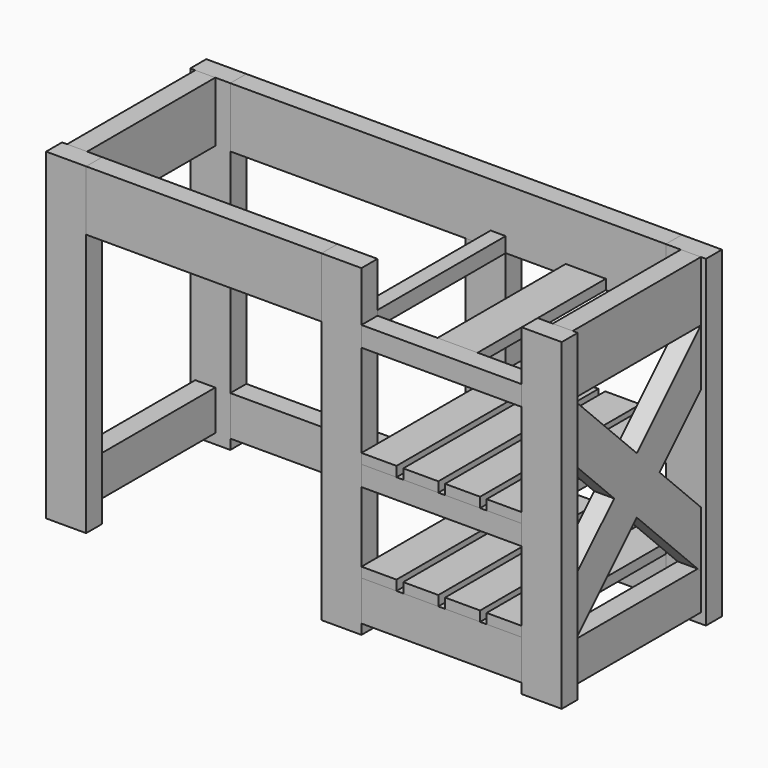
from build123d import *

# Parameters (mm, degrees)
F0_W      = 50.8
F0_H      = 819.15
F1_DEPTH  = 101.6
F2_W      = 50.8
F2_H      = 152.4
F3_DEPTH  = 406.4
F2_H_2    = 101.6
F5_DEPTH  = 50.8
F9_W      = 50.8
F9_H      = 50.8
F10_DEPTH = 406.4
F6_W      = 50.8
F6_H      = 101.6
F12_DEPTH = 1104.9
F11_W     = 50.8
F11_H     = 819.15
F13_DEPTH = 101.6
F11_H_2   = 539.75
F14_W     = 88.9
F14_H     = 25.4
F15_DEPTH = 508
F16_DEPTH = 406.4
F17_W     = 50.8
F17_H     = 152.4
F18_DEPTH = 596.9
F19_DEPTH = 1104.9
F20_W     = 101.6
F20_H     = 25.4
F21_DEPTH = 406.4
F20_W_2   = 38.0999999999
F20_H_2   = 38.1
F20_W_3   = 38.1


# Not quite as in the source:
# - a feature names something its author has since deleted; it is built from what else it names


with BuildPart() as f1:
    # F0 (on Right) → F1 (new body)
    with BuildSketch(Plane.YZ):
        with Locations((-228.6, 0)):
            Rectangle(F0_W, F0_H)
    extrude(amount=F1_DEPTH)


with BuildPart() as f1b:
    # F0 (on Right) → F1, piece 2 (new body)
    with BuildSketch(Plane.YZ):
        with Locations((228.6, 0)):
            Rectangle(F0_W, F0_H)
    extrude(amount=F1_DEPTH)


with BuildPart() as f3:
    # F2 (on face) → F3 (new body, through all)
    with BuildSketch(Plane(origin=(0, -203.2, 0), x_dir=(-1, 0, 0), z_dir=(0, 1, 0))):
        with Locations((-63.5, 333.375)):
            Rectangle(F2_W, F2_H)
    extrude(amount=F3_DEPTH)


with BuildPart() as f3b:
    # F2 (on face) → F3, piece 2 (new body, through all)
    with BuildSketch(Plane(origin=(0, -203.2, 0), x_dir=(-1, 0, 0), z_dir=(0, 1, 0))):
        with Locations((-63.5, -333.375)):
            Rectangle(F2_W, F2_H_2)
    extrude(amount=F3_DEPTH)


with BuildPart() as f5:
    # F4 (on face) → F5 (new body)
    with BuildSketch(Plane.YZ.offset(88.9)):
        Polygon((0, 53.975), (-203.2, 257.175), (-203.2, 113.4909020629), (-71.8420489686, -17.8670489685), (0, -89.7090979371), (203.2, -292.9090979371), (203.2, -149.225), (71.8420489685, -17.8670489685), align=None)
        Polygon((203.2, 257.175), (0, 53.975), (71.8420489685, -17.8670489685), (203.2, 113.4909020629), align=None)
        Polygon((0, -89.7090979371), (-71.8420489686, -17.8670489685), (-203.2, -149.225), (-203.2, -292.9090979371), align=None)
    extrude(amount=-F5_DEPTH)


with BuildPart() as f8_1:
    # F8: instance of F1b
    add(f1b.part.mirror(Plane(origin=(-552.45, -228.6, 0), x_dir=(0, 1, 0), z_dir=(-1, 0, 0))))


with BuildPart() as f8_2:
    # F8: instance of F3
    add(f3.part.mirror(Plane(origin=(-552.45, -228.6, 0), x_dir=(0, 1, 0), z_dir=(-1, 0, 0))))


with BuildPart() as f8_3:
    # F8: instance of F1
    add(f1.part.mirror(Plane(origin=(-552.45, -228.6, 0), x_dir=(0, 1, 0), z_dir=(-1, 0, 0))))


with BuildPart() as f8_4:
    # F8: instance of F3b
    add(f3b.part.mirror(Plane(origin=(-552.45, -228.6, 0), x_dir=(0, 1, 0), z_dir=(-1, 0, 0))))


with BuildPart() as f10:
    # F9 (on face) → F10 (new body)
    with BuildSketch(Plane(origin=(0, 0, 0), x_dir=(0, -1, 0), z_dir=(-1, 0, 0))):
        with Locations((228.6, 257.175)):
            Rectangle(F9_W, F9_H)
    extrude(amount=F10_DEPTH)


with BuildPart() as f10b:
    # F9 (on face) → F10, piece 2 (new body)
    with BuildSketch(Plane(origin=(0, 0, 0), x_dir=(0, -1, 0), z_dir=(-1, 0, 0))):
        with Locations((228.6, -53.975)):
            Rectangle(F9_W, F9_H)
    extrude(amount=F10_DEPTH)


with BuildPart() as f10c:
    # F9 (on face) → F10, piece 3 (new body)
    with BuildSketch(Plane(origin=(0, 0, 0), x_dir=(0, -1, 0), z_dir=(-1, 0, 0))):
        with Locations((-228.6, -53.975)):
            Rectangle(F9_W, F9_H)
    extrude(amount=F10_DEPTH)


with BuildPart() as f12:
    # F6 (on face) → F12 (new body, through all)
    with BuildSketch(Plane(origin=(0, 0, 0), x_dir=(0, -1, 0), z_dir=(-1, 0, 0))):
        with Locations((-228.6, -333.375)):
            Rectangle(F6_W, F6_H)
    extrude(amount=F12_DEPTH)


with BuildPart() as f13:
    # F11 (on face) → F13 (new body)
    with BuildSketch(Plane(origin=(-406.4, 0, 0), x_dir=(0, -1, 0), z_dir=(-1, 0, 0))):
        with Locations((228.6, 0)):
            Rectangle(F11_W, F11_H)
    extrude(amount=F13_DEPTH)


with BuildPart() as f13b:
    # F11 (on face) → F13, piece 2 (new body)
    with BuildSketch(Plane(origin=(-406.4, 0, 0), x_dir=(0, -1, 0), z_dir=(-1, 0, 0))):
        with Locations((-228.6, -12.7)):
            Rectangle(F11_W, F11_H_2)
    extrude(amount=F13_DEPTH)


with BuildPart() as f15:
    # F14 (on face) → F15 (new body, through all)
    with BuildSketch(Plane.XZ.offset(254)):
        with Locations((-44.45, -15.875)):
            Rectangle(F14_W, F14_H)
    extrude(amount=-F15_DEPTH)


with BuildPart() as f15b:
    # F14 (on face) → F15, piece 2 (new body, through all)
    with BuildSketch(Plane.XZ.offset(254)):
        with Locations((-361.95, -15.875)):
            Rectangle(F14_W, F14_H)
    extrude(amount=-F15_DEPTH)


with BuildPart() as f15c:
    # F14 (on face) → F15, piece 3 (new body, through all)
    with BuildSketch(Plane.XZ.offset(254)):
        with Locations((-255.905, -15.875)):
            Rectangle(F14_W, F14_H)
    extrude(amount=-F15_DEPTH)


with BuildPart() as f15d:
    # F14 (on face) → F15, piece 4 (new body, through all)
    with BuildSketch(Plane.XZ.offset(254)):
        with Locations((-149.86, -15.875)):
            Rectangle(F14_W, F14_H)
    extrude(amount=-F15_DEPTH)


with BuildPart() as f15e:
    # F14 (on face) → F15, piece 5 (new body, through all)
    with BuildSketch(Plane.XZ.offset(254)):
        with Locations((-44.45, -269.875)):
            Rectangle(F14_W, F14_H)
    extrude(amount=-F15_DEPTH)


with BuildPart() as f15f:
    # F14 (on face) → F15, piece 6 (new body, through all)
    with BuildSketch(Plane.XZ.offset(254)):
        with Locations((-361.95, -269.875)):
            Rectangle(F14_W, F14_H)
    extrude(amount=-F15_DEPTH)


with BuildPart() as f15g:
    # F14 (on face) → F15, piece 7 (new body, through all)
    with BuildSketch(Plane.XZ.offset(254)):
        with Locations((-255.905, -269.875)):
            Rectangle(F14_W, F14_H)
    extrude(amount=-F15_DEPTH)


with BuildPart() as f15h:
    # F14 (on face) → F15, piece 8 (new body, through all)
    with BuildSketch(Plane.XZ.offset(254)):
        with Locations((-149.86, -269.875)):
            Rectangle(F14_W, F14_H)
    extrude(amount=-F15_DEPTH)


with BuildPart() as f16:
    # F6 (on face) → F16 (new body, through all)
    with BuildSketch(Plane(origin=(0, 0, 0), x_dir=(0, -1, 0), z_dir=(-1, 0, 0))):
        with Locations((228.6, -333.375)):
            Rectangle(F6_W, F6_H)
    extrude(amount=F16_DEPTH)


with BuildPart() as f18:
    # F17 (on face) → F18 (new body, through all)
    with BuildSketch(Plane.YZ.offset(-1104.9)):
        with Locations((-228.6, 333.375)):
            Rectangle(F17_W, F17_H)
    extrude(amount=F18_DEPTH)


with BuildPart() as f19:
    # F17 (on face) → F19 (new body, through all)
    with BuildSketch(Plane.YZ.offset(-1104.9)):
        with Locations((228.6, 333.375)):
            Rectangle(F17_W, F17_H)
    extrude(amount=F19_DEPTH)


with BuildPart() as f21:
    # F20 (on face) → F21 (new body, through all)
    with BuildSketch(Plane.XZ.offset(-203.2)):
        with Locations((-203.2, 269.875)):
            Rectangle(F20_W, F20_H)
    extrude(amount=F21_DEPTH)


with BuildPart() as f21b:
    # F20 (on face) → F21, piece 2 (new body, through all)
    with BuildSketch(Plane.XZ.offset(-203.2)):
        with Locations((19.0500000001, 276.225)):
            Rectangle(F20_W_2, F20_H_2)
    extrude(amount=F21_DEPTH)


with BuildPart() as f21c:
    # F20 (on face) → F21, piece 3 (new body, through all)
    with BuildSketch(Plane.XZ.offset(-203.2)):
        with Locations((-425.45, 276.225)):
            Rectangle(F20_W_3, F20_H_2)
    extrude(amount=F21_DEPTH)


solid = Compound([f1.part, f1b.part, f3.part, f3b.part, f5.part, f8_1.part, f8_2.part, f8_3.part, f8_4.part, f10.part, f10b.part, f10c.part, f12.part, f13.part, f13b.part, f15.part, f15b.part, f15c.part, f15d.part, f15e.part, f15f.part, f15g.part, f15h.part, f16.part, f18.part, f19.part, f21.part, f21b.part, f21c.part])
